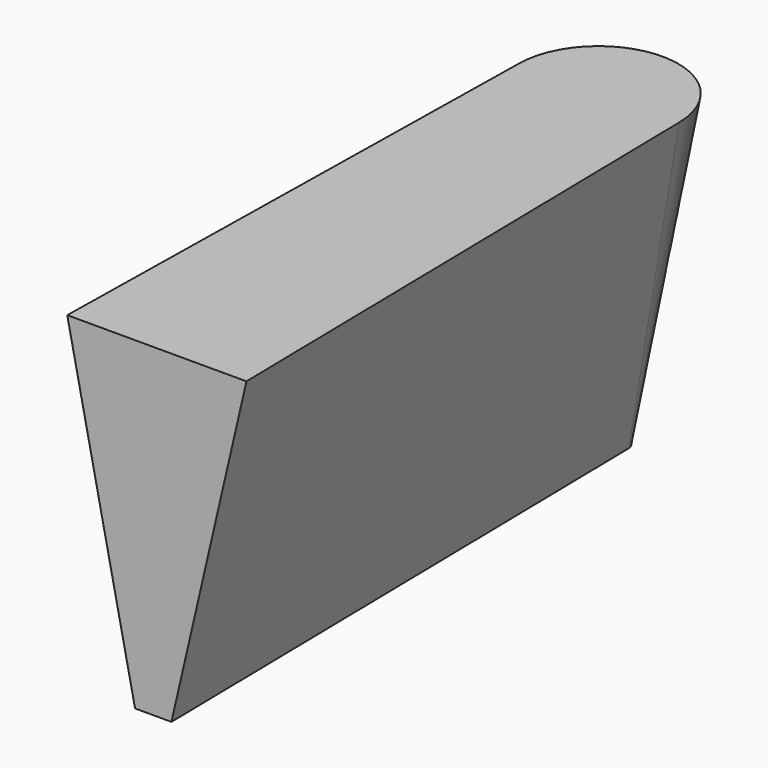
from build123d import *


# Not quite as in the source:
# - ends of sketch curves that miss each other by under 0.0002 mm in the source are joined


with BuildPart() as f3:
    # F1 (on offset) → F3 section 0
    with BuildSketch(Plane.XY.offset(152.4)):
        with BuildLine():
            Line((-42.50436, -194.0035744), (42.50436, -194.0035744))
            Line((42.50436, -194.0035744), (37.9258068, 68.301743))
            ThreePointArc((37.9258068, 68.301743), (0, 105.809161), (-37.9258100359, 68.3017430359))
            Line((-37.9258100359, 68.3017430359), (-42.50436, -194.0035744))
        make_face()
    # F2 (on Top) → F3 section 1
    with BuildSketch(Plane.XY):
        with BuildLine():
            Line((-3.7925756, 81.1910746), (-8.63346, -196.1422544))
            Line((-8.63346, -196.1422544), (8.63346, -196.1422544))
            Line((8.63346, -196.1422544), (3.7925756, 81.1910746))
            ThreePointArc((3.7925756, 81.1910746), (0, 84.9758778), (-3.7925756, 81.1910746))
        make_face()
    loft()


solid = f3.part
